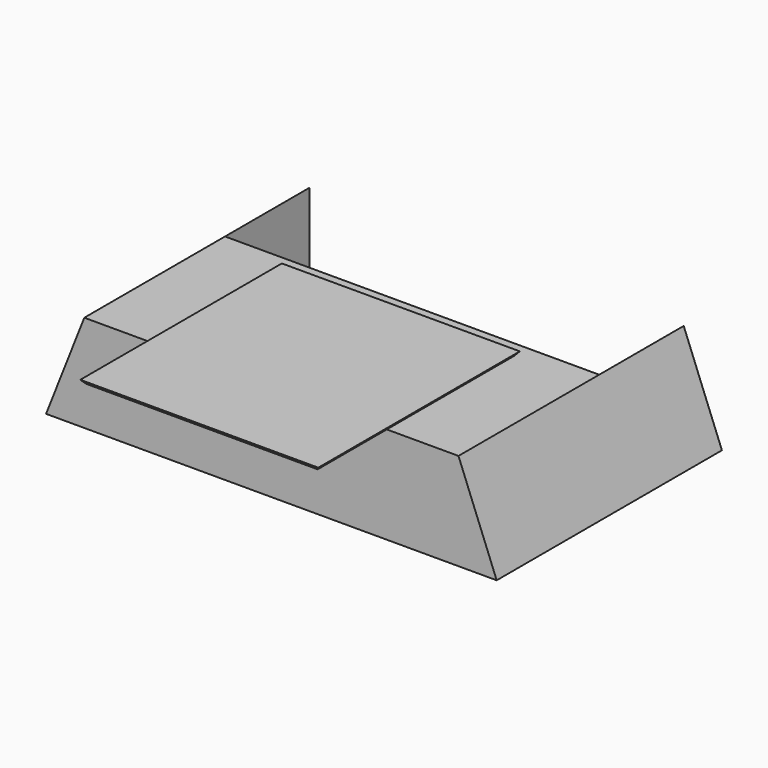
from build123d import *

# Parameters (mm, degrees)
F0_W     = 48.9477626979
F0_H     = 23.0111181736
F1_DEPTH = 12.7
F3_DEPTH = 36.83
F4_W     = 30.2896779031
F4_H     = 32.1149742231
F5_DEPTH = 0.5
F5_TAPER = -40


# Not quite as in the source:
# - the program builds the solid bodies; features that only make, move or delete a surface that nothing else refers to are left out


with BuildPart() as f1:
    # F0 (on Top) → F1 (new body)
    with BuildSketch(Plane.XY):
        with Locations((0, -11.5055590868)):
            Rectangle(F0_W, F0_H)
    extrude(amount=F1_DEPTH)

    # F2 (on face) → F3 (join)
    with BuildSketch(Plane.XZ.offset(23.0111181736)):
        Polygon((29.4724665582, 0), (24.473881349, 12.7), (24.473881349, 0), align=None)
        Polygon((-24.473881349, 0), (-24.473881349, 12.7), (-29.4724665582, 0), align=None)
    extrude(amount=-F3_DEPTH)

    # F4 (on face) → F5 (join)
    with BuildSketch(Plane.XY.offset(12.7)):
        with Locations((-0.0495417044, -18.2598386891)):
            Rectangle(F4_W, F4_H)
    extrude(amount=F5_DEPTH, taper=F5_TAPER)


solid = f1.part
